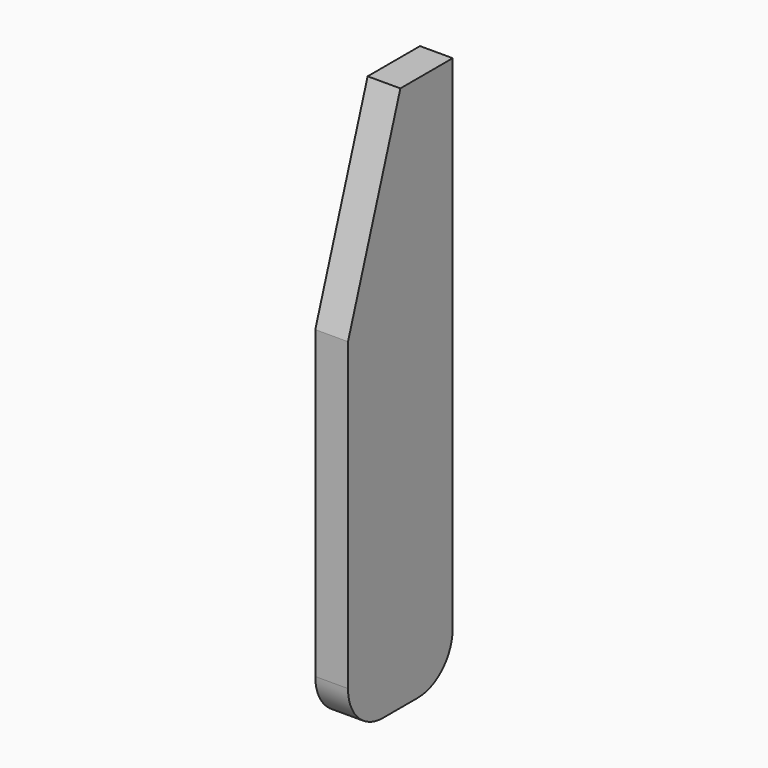
from build123d import *

# Parameters (mm, degrees)
F1_DEPTH = 9.525
F2_R     = 12.7


# Not quite as in the source:
# - a feature names something its author has since deleted; it is built from what else it names


with BuildPart() as f1:
    # F0 (on Right) → F1 (new body)
    with BuildSketch(Plane.YZ):
        Polygon((-19.05, 22.225), (-19.05, -79.375), (19.05, -79.375), (19.05, 79.375), (0, 79.375), align=None)
    extrude(amount=F1_DEPTH)

    # F2
    f2_edges = [f1.edges().sort_by_distance(p)[0] for p in [
        (4.7625, -19.05, -79.375),
        (4.7625, 19.05, -79.375),
    ]]
    fillet(f2_edges, radius=F2_R)


solid = f1.part
